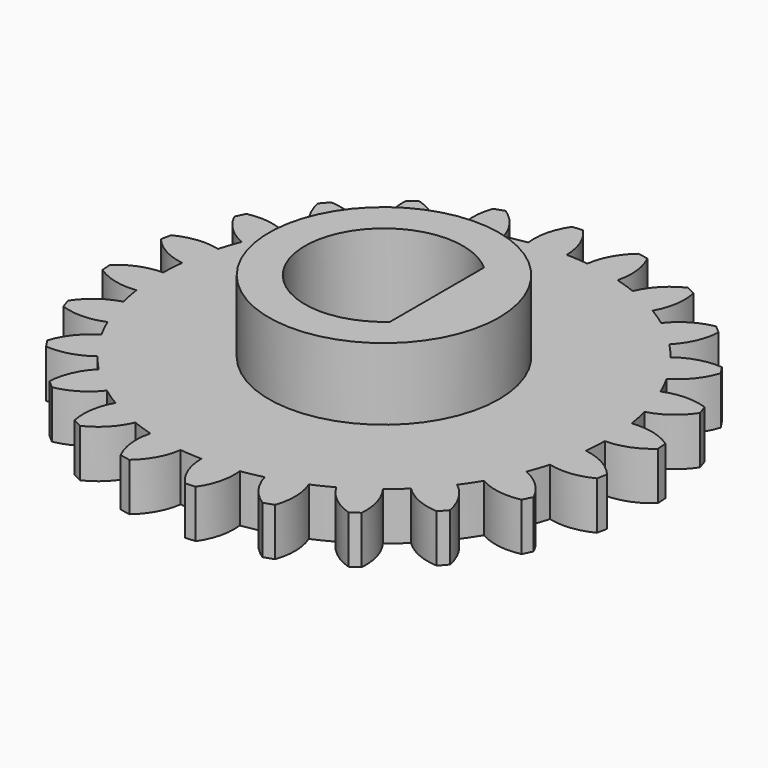
from build123d import *

# Parameters (mm, degrees)
F0_R     = 4.8
F1_DEPTH = 2
F2_DEPTH = 2
F3_COUNT = 24
F4_DEPTH = 5


# Not quite as in the source:
# - a feature names something its author has since deleted; it is built from what else it names


with BuildPart() as f1:
    # F0 (on Top) → F1 (new body)
    with BuildSketch(Plane.XY):
        with BuildLine():
            ThreePointArc((-1.3706276856, 9.2356996308), (-6.0983367739, -7.07015251), (9.33685, 0))
            ThreePointArc((9.33685, 0), (6.6561644626, 6.547689865), (0.1534010705, 9.3355897529))
            ThreePointArc((0.1534010705, 9.3355897529), (-0.6106592072, 9.3168590874), (-1.3706276856, 9.2356996308))
        make_face()
        Circle(F0_R, mode=Mode.SUBTRACT)
        Circle(F0_R)
        with BuildLine():
            ThreePointArc((2.2121703696, -2.4487348276), (-3.3, 0), (2.2121703696, 2.4487348276))
            Line((2.2121703696, 2.4487348276), (2.2121703696, -2.4487348276))
        make_face(mode=Mode.SUBTRACT)
    extrude(amount=F1_DEPTH)



with BuildPart() as f2:
    # F0 (on Top) → F2 (new body)
    with BuildSketch(Plane.XY):
        with BuildLine():
            ThreePointArc((-1.3706276856, 9.2356996308), (-0.6106592072, 9.3168590874), (0.1534010705, 9.3355897529))
            ThreePointArc((0.1534010705, 9.3355897529), (-0.020381392, 10.2397788889), (-0.5045147629, 11.0229603603))
            Line((-0.5045147629, 11.0229603603), (-0.9385864737, 10.9945097972))
            ThreePointArc((-0.9385864737, 10.9945097972), (-1.3163523212, 10.1548364665), (-1.3706276856, 9.2356996308))
        make_face()
    extrude(amount=F2_DEPTH)


with BuildPart() as f1_1:
    add(f1.part)

    add(f2.part)  # F3 merges F2
    # F3: F2 ×24 about axis
    f3_axis = Axis((0, 0, 0), (0, 0, -1))
    for i in range(1, F3_COUNT):
        add(f2.part.rotate(f3_axis, i * 360 / F3_COUNT))

    # F0 (on Top) → F4 (join)
    with BuildSketch(Plane.XY):
        Circle(F0_R)
        with BuildLine():
            ThreePointArc((2.2121703696, -2.4487348276), (-3.3, 0), (2.2121703696, 2.4487348276))
            Line((2.2121703696, 2.4487348276), (2.2121703696, -2.4487348276))
        make_face(mode=Mode.SUBTRACT)
    extrude(amount=F4_DEPTH)


solid = f1_1.part
